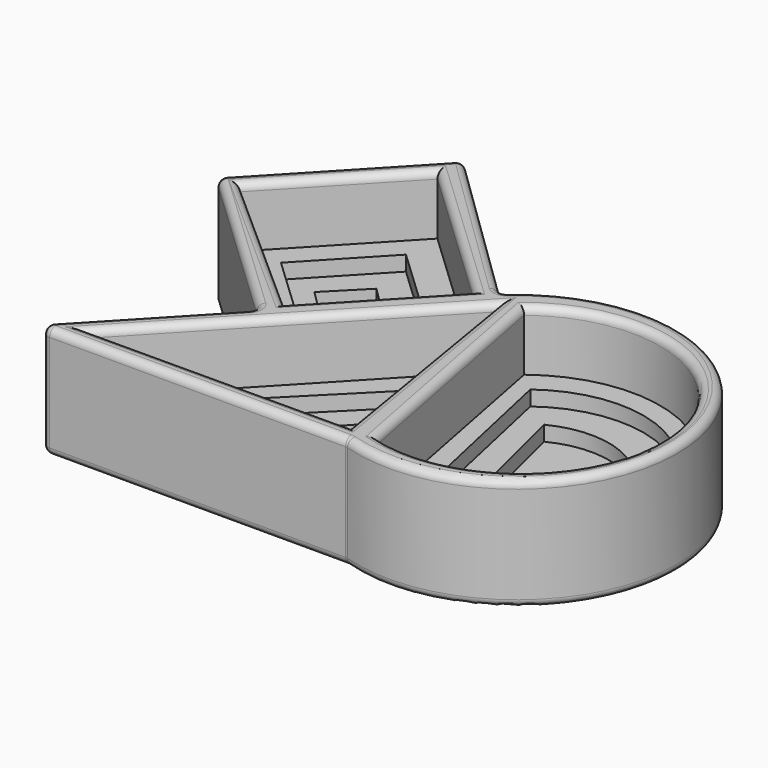
from build123d import *

# Parameters (mm, degrees)
F1_DEPTH  = 15
F3_DEPTH  = 8
F4_R      = 1
F6_DEPTH  = 2
F8_DEPTH  = 2
F10_DEPTH = 2
F12_DEPTH = 2


# Not quite as in the source:
# - a feature names something its author has since deleted; it is built from what else it names


with BuildPart() as f1:
    # F0 (on Top) → F1 (new body)
    with BuildSketch(Plane.XY):
        with BuildLine():
            Line((-28.3214918106, 39.0464443552), (-46.1799150741, 20.1475579913))
            Line((-46.1799150741, 20.1475579913), (-24.1265251153, -0.6917001902))
            Line((-24.1265251153, -0.6917001902), (-40.4306314886, -17.9457124323))
            Line((-40.4306314886, -17.9457124323), (1.5834453516, -17.9457124323))
            ThreePointArc((1.5834453516, -17.9457124323), (28.9057292456, 7.2125327526), (-6.6504706629, 17.9457124323))
            Line((-6.6504706629, 17.9457124323), (-28.3214918106, 39.0464443552))
        make_face()
    extrude(amount=F1_DEPTH)

    # F2 (on face) → F3 (cut)
    with BuildSketch(Plane.XY.offset(15)):
        with BuildLine():
            Line((-2.5950646959, 16.9163886458), (3.7065453362, -15.5357513577))
            ThreePointArc((3.7065453362, -15.5357513577), (26.9474296129, 5.8151003686), (-2.5950646959, 16.9163886458))
        make_face()
        Polygon((-5.1901293918, 15.8294621167), (-34.8258907848, -15.5329307781), (0, -15.4121983796), align=None)
        Polygon((-28.8714991264, 35.28469053), (-43.1752689183, 20.1475579913), (-22.7079026012, 1.9694547007), (-8.9844264049, 16.4924847199), align=None)
    extrude(amount=-F3_DEPTH, mode=Mode.SUBTRACT)

    # F4
    f4_edges = [f1.edges().sort_by_distance(p)[0] for p in [
        (-37.250703, 29.597001, 0),
        (-35.15322, 9.727929, 0),
        (-32.278578, -9.318706, 0),
        (-19.423593, -17.945712, 0),
        (28.905729, 7.212533, 0),
        (-17.485981, 28.496078, 0),
        (-18.927963, 25.888588, 15),
        (-36.023384, 27.716124, 15),
        (-32.941586, 11.058506, 15),
        (-15.846165, 9.23097, 15),
        (-17.412945, -15.472565, 15),
        (-20.00801, 0.148266, 15),
        (-2.595065, 0.208632, 15),
        (0.55574, 0.690319, 15),
        (26.94743, 5.8151, 15),
        (28.905729, 7.212533, 15),
        (-19.423593, -17.945712, 15),
        (-32.278578, -9.318706, 15),
        (-35.15322, 9.727929, 15),
        (-37.250703, 29.597001, 15),
        (-17.485981, 28.496078, 15),
        (-6.650471, 17.945712, 7.5),
        (-28.321492, 39.046444, 7.5),
        (-46.179915, 20.147558, 7.5),
        (-40.430631, -17.945712, 7.5),
        (-24.126525, -0.6917, 7.5),
        (1.583445, -17.945712, 7.5),
    ]]
    fillet(f4_edges, radius=F4_R)

    # F5 (on face) → F6 (cut)
    with BuildSketch(Plane.XY.offset(7)):
        Polygon((-29.1725099087, -12.9052552501), (-3.2478775829, -12.3988948762), (-7.4992091395, 8.8786818087), align=None)
        Polygon((-23.3146349898, 6.744285012), (-14.0517026385, 16.1163697069), (-29.1725099087, 30.4047130048), (-38.2205257573, 20.8295438638), align=None)
        with BuildLine():
            Line((0, 14.7073501721), (6.1764790816, -13.333094822))
            ThreePointArc((6.1764790816, -13.333094822), (24.8870467759, 5.4887589231), (0, 14.7073501721))
        make_face()
    extrude(amount=-F6_DEPTH, mode=Mode.SUBTRACT)

    # F7 (on face) → F8 (cut)
    with BuildSketch(Plane.XY.offset(5)):
        with BuildLine():
            Line((3.6986530758, 12.4016236514), (9.2264488339, -9.847166948))
            ThreePointArc((9.2264488339, -9.847166948), (20.4226323137, 4.7456631043), (3.6986530758, 12.4016236514))
        make_face()
    extrude(amount=-F8_DEPTH, mode=Mode.SUBTRACT)

    # F9 (on face) → F10 (cut)
    with BuildSketch(Plane.XY.offset(5)):
        Polygon((-9.698738344, 2.2434238344), (-19.8120251298, -8.6724534631), (-7.6682440939, -8.4352609186), align=None)
    extrude(amount=-F10_DEPTH, mode=Mode.SUBTRACT)

    # F11 (on face) → F12 (cut)
    with BuildSketch(Plane.XY.offset(5)):
        Polygon((-33.7495236595, 20.8295438638), (-23.5399451314, 10.7388715832), (-18.9629313805, 15.3698198505), (-29.1725099087, 25.4604921311), align=None)
    extrude(amount=-F12_DEPTH, mode=Mode.SUBTRACT)


solid = f1.part
